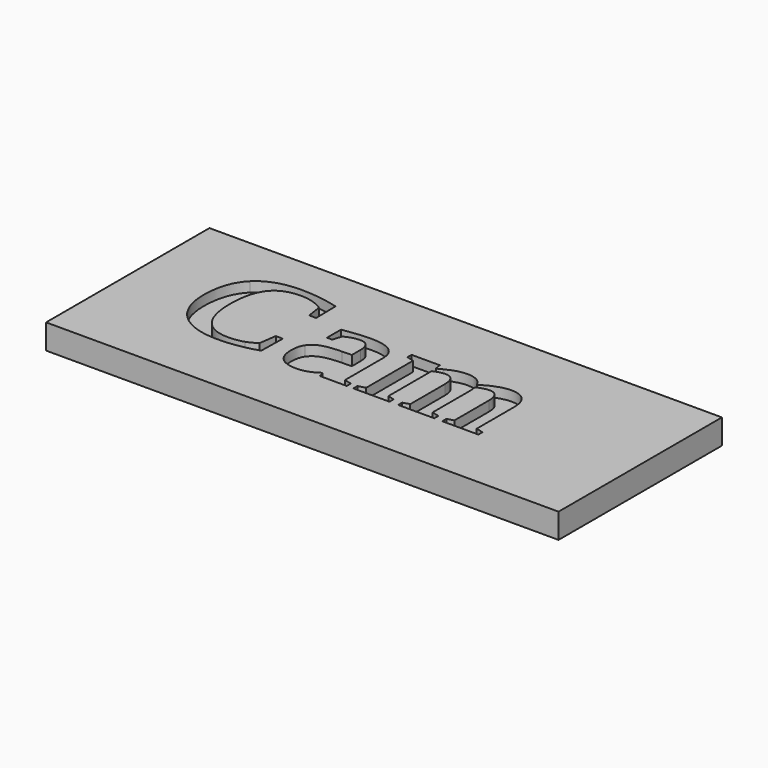
from build123d import *

# Parameters (mm, degrees)
F0_W     = 102.9875054955
F0_H     = 41.0375036299
F1_DEPTH = 3
F2_W     = 102.9875054955
F2_H     = 41.0375036299
F3_DEPTH = 2


with BuildPart() as f1:
    # F0 (on Top) → F1 (new body)
    with BuildSketch(Plane.XY):
        with Locations((-51.4937527478, -20.518751815)):
            Rectangle(F0_W, F0_H)
    extrude(amount=F1_DEPTH)

    # F2 (on face) → F3 (join)
    with BuildSketch(Plane.XY.offset(3)):
        with Locations((-51.4937527478, -20.518751815)):
            Rectangle(F2_W, F2_H)
        with BuildLine():
            add(Edge.make_bspline(
                [(-61.8547136732, -13.5894833709), (-60.7502540071, -13.4974450654), (-59.601018949, -13.4974450654)],
                knots=[0, 0, 0, 1, 1, 1], degree=2))
            add(Edge.make_bspline(
                [(-59.601018949, -13.4974450654), (-54.1135459231, -13.4974450654), (-54.1135459231, -17.5371804208)],
                knots=[0, 0, 0, 1, 1, 1], degree=2))
            Line((-54.1135459231, -17.5371804208), (-54.1135459231, -27.0395135845))
            Line((-54.1135459231, -27.0395135845), (-52.650883122, -27.4126418501))
            Line((-52.650883122, -27.4126418501), (-52.650883122, -28.4375008196))
            Line((-52.650883122, -28.4375008196), (-58.02890519, -28.4375008196))
            Line((-58.02890519, -28.4375008196), (-58.3721831944, -27.3181160228))
            add(Edge.make_bspline(
                [(-58.3721831944, -27.3181160228), (-59.5860938184, -28.1439732506), (-60.5636898743, -28.4474509066)],
                knots=[0, 0, 0, 1, 1, 1], degree=2))
            add(Edge.make_bspline(
                [(-60.5636898743, -28.4474509066), (-61.5412859301, -28.7509285627), (-62.5362946383, -28.7509285627)],
                knots=[0, 0, 0, 1, 1, 1], degree=2))
            add(Edge.make_bspline(
                [(-62.5362946383, -28.7509285627), (-67.0635842608, -28.7509285627), (-67.0635842608, -24.3927904206)],
                knots=[0, 0, 0, 1, 1, 1], degree=2))
            add(Edge.make_bspline(
                [(-67.0635842608, -24.3927904206), (-67.0635842608, -22.7460510085), (-66.3944409045, -21.7585048655)],
                knots=[0, 0, 0, 1, 1, 1], degree=2))
            add(Edge.make_bspline(
                [(-66.3944409045, -21.7585048655), (-65.7252975482, -20.7709587226), (-64.4666115323, -20.2983295862)],
                knots=[0, 0, 0, 1, 1, 1], degree=2))
            add(Edge.make_bspline(
                [(-64.4666115323, -20.2983295862), (-63.2079255164, -19.8257004498), (-60.50150183, -19.7610248837)],
                knots=[0, 0, 0, 1, 1, 1], degree=2))
            Line((-60.50150183, -19.7610248837), (-58.6060102408, -19.7162494919))
            Line((-58.6060102408, -19.7162494919), (-58.6060102408, -17.5869308562))
            add(Edge.make_bspline(
                [(-58.6060102408, -17.5869308562), (-58.6060102408, -14.9402076923), (-60.7651791377, -14.9402076923)],
                knots=[0, 0, 0, 1, 1, 1], degree=2))
            add(Edge.make_bspline(
                [(-60.7651791377, -14.9402076923), (-62.073615589, -14.9402076923), (-63.6905047399, -15.7511397895)],
                knots=[0, 0, 0, 1, 1, 1], degree=2))
            Line((-63.6905047399, -15.7511397895), (-64.2775598778, -17.5720057256))
            Line((-64.2775598778, -17.5720057256), (-65.3073938908, -17.5720057256))
            Line((-65.3073938908, -17.5720057256), (-65.3073938908, -14.0397248114))
            add(Edge.make_bspline(
                [(-65.3073938908, -14.0397248114), (-62.9591733393, -13.6815216764), (-61.8547136732, -13.5894833709)],
                knots=[0, 0, 0, 1, 1, 1], degree=2))
        make_face(mode=Mode.SUBTRACT)
        with BuildLine():
            Line((-45.6360717289, -13.8208228956), (-45.4221448567, -15.0994090857))
            Line((-45.4221448567, -15.0994090857), (-44.3624605824, -14.5521542961))
            add(Edge.make_bspline(
                [(-44.3624605824, -14.5521542961), (-42.1883665549, -13.4327694994), (-40.4620264461, -13.4327694994)],
                knots=[0, 0, 0, 1, 1, 1], degree=2))
            add(Edge.make_bspline(
                [(-40.4620264461, -13.4327694994), (-37.850128587, -13.4327694994), (-36.9794959673, -15.3332361321)],
                knots=[0, 0, 0, 1, 1, 1], degree=2))
            add(Edge.make_bspline(
                [(-36.9794959673, -15.3332361321), (-33.7904930574, -13.4327694994), (-31.6014738993, -13.4327694994)],
                knots=[0, 0, 0, 1, 1, 1], degree=2))
            add(Edge.make_bspline(
                [(-31.6014738993, -13.4327694994), (-27.6512893276, -13.4327694994), (-27.6512893276, -17.741157206)],
                knots=[0, 0, 0, 1, 1, 1], degree=2))
            Line((-27.6512893276, -17.741157206), (-27.6512893276, -27.0395135845))
            Line((-27.6512893276, -27.0395135845), (-26.1886265265, -27.4126418501))
            Line((-26.1886265265, -27.4126418501), (-26.1886265265, -28.4375008196))
            Line((-26.1886265265, -28.4375008196), (-33.4472150531, -28.4375008196))
            Line((-33.4472150531, -28.4375008196), (-33.4472150531, -27.4126418501))
            Line((-33.4472150531, -27.4126418501), (-32.1437536453, -27.0395135845))
            Line((-32.1437536453, -27.0395135845), (-32.1437536453, -18.348112518))
            add(Edge.make_bspline(
                [(-32.1437536453, -18.348112518), (-32.1437536453, -17.0396760667), (-32.6487205647, -16.3108321879)],
                knots=[0, 0, 0, 1, 1, 1], degree=2))
            add(Edge.make_bspline(
                [(-32.6487205647, -16.3108321879), (-33.1536874841, -15.5819883091), (-34.1785464536, -15.5819883091)],
                knots=[0, 0, 0, 1, 1, 1], degree=2))
            add(Edge.make_bspline(
                [(-34.1785464536, -15.5819883091), (-35.3327565552, -15.5819883091), (-36.6660682242, -16.233719013)],
                knots=[0, 0, 0, 1, 1, 1], degree=2))
            add(Edge.make_bspline(
                [(-36.6660682242, -16.233719013), (-36.5118418744, -16.8854497169), (-36.5118418744, -17.741157206)],
                knots=[0, 0, 0, 1, 1, 1], degree=2))
            Line((-36.5118418744, -17.741157206), (-36.5118418744, -27.0395135845))
            Line((-36.5118418744, -27.0395135845), (-35.0491790733, -27.4126418501))
            Line((-35.0491790733, -27.4126418501), (-35.0491790733, -28.4375008196))
            Line((-35.0491790733, -28.4375008196), (-42.3127426434, -28.4375008196))
            Line((-42.3127426434, -28.4375008196), (-42.3127426434, -27.4126418501))
            Line((-42.3127426434, -27.4126418501), (-41.0043061921, -27.0395135845))
            Line((-41.0043061921, -27.0395135845), (-41.0043061921, -18.348112518))
            add(Edge.make_bspline(
                [(-41.0043061921, -18.348112518), (-41.0043061921, -17.0396760667), (-41.5092731115, -16.3108321879)],
                knots=[0, 0, 0, 1, 1, 1], degree=2))
            add(Edge.make_bspline(
                [(-41.5092731115, -16.3108321879), (-42.014240031, -15.5819883091), (-43.0415865222, -15.5819883091)],
                knots=[0, 0, 0, 1, 1, 1], degree=2))
            add(Edge.make_bspline(
                [(-43.0415865222, -15.5819883091), (-44.0689330135, -15.5819883091), (-45.3873195519, -16.1839685776)],
                knots=[0, 0, 0, 1, 1, 1], degree=2))
            Line((-45.3873195519, -16.1839685776), (-45.3873195519, -27.0395135845))
            Line((-45.3873195519, -27.0395135845), (-44.0540078829, -27.4126418501))
            Line((-44.0540078829, -27.4126418501), (-44.0540078829, -28.4375008196))
            Line((-44.0540078829, -28.4375008196), (-51.3125964094, -28.4375008196))
            Line((-51.3125964094, -28.4375008196), (-51.3125964094, -27.4126418501))
            Line((-51.3125964094, -27.4126418501), (-49.8847589131, -27.0395135845))
            Line((-49.8847589131, -27.0395135845), (-49.8847589131, -15.2237851742))
            Line((-49.8847589131, -15.2237851742), (-51.3125964094, -14.8506569086))
            Line((-51.3125964094, -14.8506569086), (-51.3125964094, -13.8208228956))
            Line((-51.3125964094, -13.8208228956), (-45.6360717289, -13.8208228956))
        make_face(mode=Mode.SUBTRACT)
        with BuildLine():
            add(Edge.make_bspline(
                [(-74.2475471343, -28.36785021), (-76.4863167278, -28.7509285627), (-78.4116585783, -28.7509285627)],
                knots=[0, 0, 0, 1, 1, 1], degree=2))
            add(Edge.make_bspline(
                [(-78.4116585783, -28.7509285627), (-83.6503794271, -28.7509285627), (-86.5881426382, -25.9673917014)],
                knots=[0, 0, 0, 1, 1, 1], degree=2))
            add(Edge.make_bspline(
                [(-86.5881426382, -25.9673917014), (-89.5259058493, -23.1838548401), (-89.5259058493, -18.2535866908)],
                knots=[0, 0, 0, 1, 1, 1], degree=2))
            add(Edge.make_bspline(
                [(-89.5259058493, -18.2535866908), (-89.5259058493, -12.905414884), (-86.719981292, -10.129340588)],
                knots=[0, 0, 0, 1, 1, 1], degree=2))
            add(Edge.make_bspline(
                [(-86.719981292, -10.129340588), (-83.9140567348, -7.353266292), (-78.4265837089, -7.353266292)],
                knots=[0, 0, 0, 1, 1, 1], degree=2))
            add(Edge.make_bspline(
                [(-78.4265837089, -7.353266292), (-74.8047520109, -7.353266292), (-70.9192430052, -8.3980254357)],
                knots=[0, 0, 0, 1, 1, 1], degree=2))
            Line((-70.9192430052, -8.3980254357), (-70.824717178, -13.4029192381))
            Line((-70.824717178, -13.4029192381), (-72.222704413, -13.4029192381))
            Line((-72.222704413, -13.4029192381), (-72.6605082447, -10.3880428522))
            add(Edge.make_bspline(
                [(-72.6605082447, -10.3880428522), (-74.7102261836, -8.9900556171), (-77.4315750006, -8.9900556171)],
                knots=[0, 0, 0, 1, 1, 1], degree=2))
            add(Edge.make_bspline(
                [(-77.4315750006, -8.9900556171), (-81.038481568, -8.9900556171), (-82.7026336325, -11.2362877759)],
                knots=[0, 0, 0, 1, 1, 1], degree=2))
            add(Edge.make_bspline(
                [(-82.7026336325, -11.2362877759), (-84.3667856971, -13.4825199348), (-84.3667856971, -18.2088112989)],
                knots=[0, 0, 0, 1, 1, 1], degree=2))
            add(Edge.make_bspline(
                [(-84.3667856971, -18.2088112989), (-84.3667856971, -22.5768995281), (-82.6255204576, -24.8629320352)],
                knots=[0, 0, 0, 1, 1, 1], degree=2))
            add(Edge.make_bspline(
                [(-82.6255204576, -24.8629320352), (-80.8842552182, -27.1489645424), (-77.5559510892, -27.1489645424)],
                knots=[0, 0, 0, 1, 1, 1], degree=2))
            add(Edge.make_bspline(
                [(-77.5559510892, -27.1489645424), (-75.7997607191, -27.1489645424), (-74.4863492243, -26.6813104495)],
                knots=[0, 0, 0, 1, 1, 1], degree=2))
            add(Edge.make_bspline(
                [(-74.4863492243, -26.6813104495), (-73.1729377294, -26.2136563567), (-72.4266811982, -25.5768507834)],
                knots=[0, 0, 0, 1, 1, 1], degree=2))
            Line((-72.4266811982, -25.5768507834), (-71.9291768441, -22.1540208271))
            Line((-71.9291768441, -22.1540208271), (-70.5162644784, -22.1540208271))
            Line((-70.5162644784, -22.1540208271), (-70.6058152621, -27.4424921113))
            add(Edge.make_bspline(
                [(-70.6058152621, -27.4424921113), (-72.0087775408, -27.9847718573), (-74.2475471343, -28.36785021)],
                knots=[0, 0, 0, 1, 1, 1], degree=2))
        make_face(mode=Mode.SUBTRACT)
    extrude(amount=F3_DEPTH)


solid = f1.part
